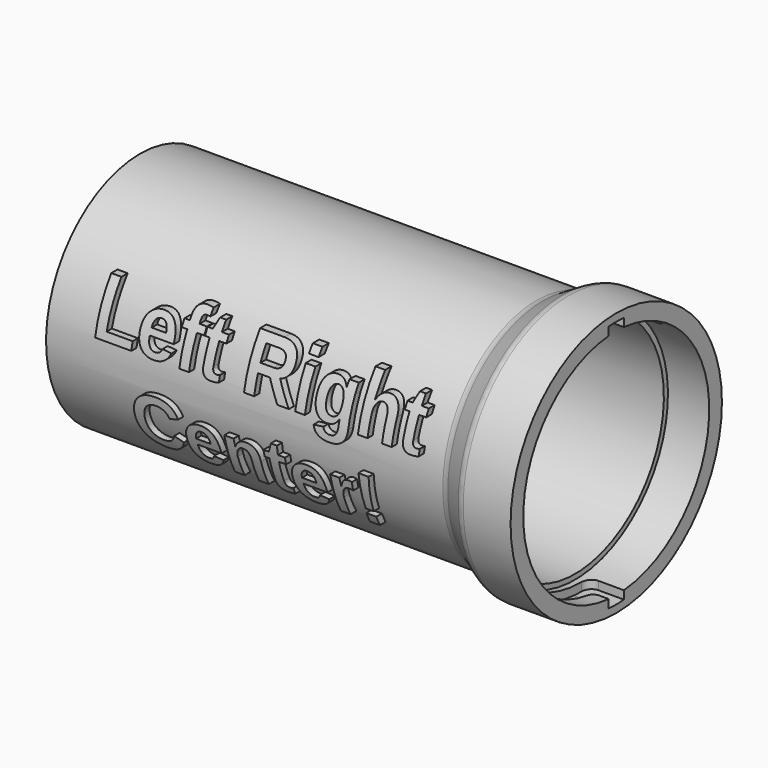
from build123d import *

# Parameters (mm, degrees)
F2_R          = 2
F4_DEPTH      = 5.5
F5_W          = 3
F5_H          = 7.349659
F6_ANGLE      = 45
F7_W          = 3
F7_H          = 8.315017
F8_ANGLE      = 45
F9_R          = 1.5
F10_R         = 1.49999
F11_R         = 1
F13_TEXT_SIZE = 11.111111
F14_DEPTH     = 20
F15_R         = 24.5
F15_R_2       = 19.5
F16_DEPTH     = 61.2
F17_DEPTH     = 74.001


# Not quite as in the source:
# - a fillet or chamfer is up to 0.001 mm smaller than in the source, because OpenCascade refuses the exact size
# - Text() gives the source's letters only with a copy of the font that has no kerning and outlines rounded to 1/6400 em; it was checked with that copy


with BuildPart() as f1:
    # F0 (on Front) → F1 (revolve)
    with BuildSketch(Plane.XZ):
        Polygon((0, 18.5), (0, 0), (1, 0), (1, 17.5), (68.5, 17.5), (68.5, 18.3), (75, 18.3), (75, 20.8), (67, 20.8), (63.016283, 18.5), align=None)
    revolve(axis=Axis((0.5, 0, 0), (-1, 0, 0)))

    # F2
    f2_edges = [f1.edges().sort_by_distance(p)[0] for p in [
        (67, 0, -20.8),
        (63.016283, 0, -18.5),
    ]]
    fillet(f2_edges, radius=F2_R)

    # F3 (on face) → F4 (cut)
    with BuildSketch(Plane.YZ.offset(75)):
        with BuildLine():
            Line((1.5, -19.542518), (1.5, 19.542518))
            ThreePointArc((1.5, 19.542518), (0, 19.6), (-1.5, 19.542518))
            Line((-1.5, 19.542518), (-1.5, -19.542518))
            ThreePointArc((-1.5, -19.542518), (0, -19.6), (1.5, -19.542518))
        make_face()
    extrude(amount=-F4_DEPTH, mode=Mode.SUBTRACT)

    # F5 (on Front) → F6 (revolve, cut)
    with BuildSketch(Plane.XZ):
        with Locations((71, 15.92517)):
            Rectangle(F5_W, F5_H)
    revolve(axis=Axis((71, 0, 0), (-1, 0, 0)), revolution_arc=F6_ANGLE, mode=Mode.SUBTRACT)

    # F7 (on Front) → F8 (revolve, cut)
    with BuildSketch(Plane.XZ):
        with Locations((71, -15.442491)):
            Rectangle(F7_W, F7_H)
    revolve(axis=Axis((71, 0, 0), (-1, 0, 0)), revolution_arc=F8_ANGLE, mode=Mode.SUBTRACT)

    # F9
    f9_edges = [f1.edges().sort_by_distance(p)[0] for p in [
        (69.5, -1.5, 18.890469),
        (69.5, 1.5, -18.890469),
    ]]
    fillet(f9_edges, radius=F9_R)

    # F10 (radius 1.5 in the source; OpenCascade refuses exactly that, so slightly less here)
    f10_edges = [f1.edges().sort_by_distance(p)[0] for p in [
        (69.5, 13.399674, 13.399674),
        (72.5, 13.399674, 13.399674),
        (69.5, -13.399674, -13.399674),
        (72.5, -13.399674, -13.399674),
    ]]
    fillet(f10_edges, radius=F10_R)

    # F11
    f11_edges = [f1.edges().sort_by_distance(p)[0] for p in [
        (72.5, 1.5, 18.890469),
        (72.5, -1.5, -18.890469),
    ]]
    fillet(f11_edges, radius=F11_R)

    # F13 (on Front) → F14 (join)
    with BuildSketch(Plane.XZ):
        with Locations((7.529514, 3.5)):
            Text('Left Right', F13_TEXT_SIZE, font='Arimo', font_style=FontStyle.BOLD, text_align=(TextAlign.LEFT, TextAlign.BOTTOM))
        with Locations((13.703125, -9.277778)):
            Text('Center!', F13_TEXT_SIZE, font='Arimo', font_style=FontStyle.BOLD, text_align=(TextAlign.LEFT, TextAlign.BOTTOM))
    extrude(amount=F14_DEPTH)

    # F15 (on face) → F16 (cut)
    with BuildSketch(Plane(origin=(0, 0, 0), x_dir=(0, -1, 0), z_dir=(-1, 0, 0))):
        Circle(F15_R)
        Circle(F15_R_2, mode=Mode.SUBTRACT)
    extrude(amount=-F16_DEPTH, mode=Mode.SUBTRACT)

    # F17 (cut, through all): a face of the model
    f17_faces = [f1.faces().sort_by_distance(p)[0] for p in [
        (1, 0, 0),
    ]]
    extrude(f17_faces, amount=F17_DEPTH, mode=Mode.SUBTRACT)


solid = f1.part
